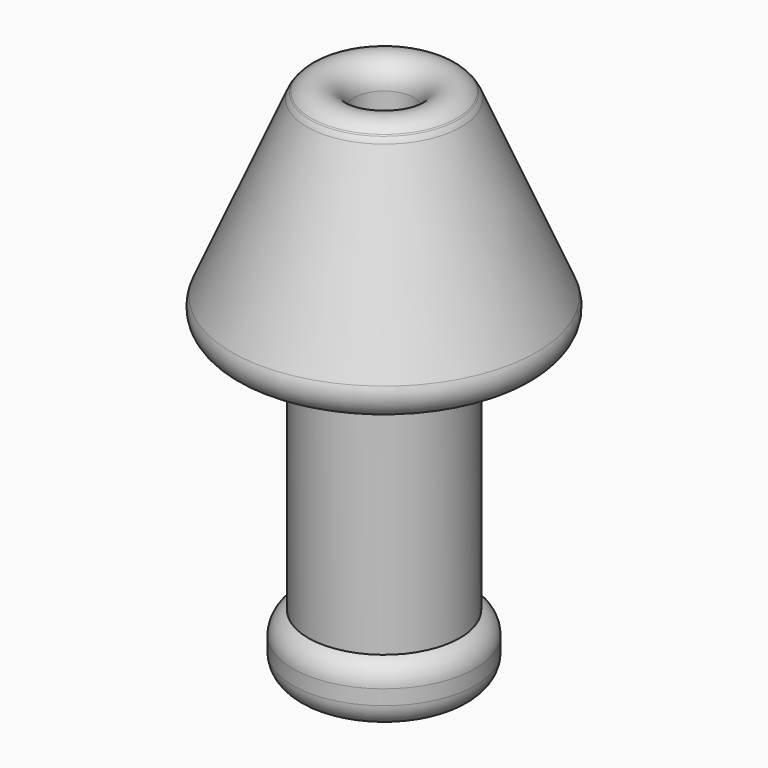
from build123d import *

# Parameters (mm, degrees)
F0_W = 0.5
F0_H = 2


# Not quite as in the source:
# - a fillet or chamfer that OpenCascade refuses, or shapes differently, is made with other operations: its cross-section is extruded or revolved along the edge and cut away or added


with BuildPart() as f1:
    # F0 (on Front) → F1 (revolve)
    with BuildSketch(Plane.XZ):
        Polygon((-2.5, 0), (-1, 0), (-1, 18.7049116939), (-2.5, 16.9229302555), (-5.5, 10), (-2.5, 10), (-2.5, 2), align=None)
        with Locations((-2.75, 1)):
            Rectangle(F0_W, F0_H)
    revolve(axis=Axis((0, 0, 13.3904740214), (0, 0, 1)))

    # F2: fillet of radius 0.8 on 5 edges, made by hand

    # F2_s1 → F2_t2 (revolve, cut)
    with BuildSketch(Plane.XZ):
        with BuildLine():
            ThreePointArc((-2.424695214, 17.0126243355), (-2.4928760132, 16.918520212), (-2.546704077, 16.8155311495))
            Line((-2.546704077, 16.8155311495), (-2.5613849178, 16.821892982))
            ThreePointArc((-2.5613849178, 16.821892982), (-2.5379640629, 16.8755627139), (-2.5146808408, 16.929292088))
            Line((-2.5146808408, 16.929292088), (-2.5122406636, 16.9332339517))
            ThreePointArc((-2.5122406636, 16.9332339517), (-2.4745308925, 16.9780326932), (-2.4369358776, 17.0229280317))
            Line((-2.4369358776, 17.0229280317), (-2.424695214, 17.0126243355))
        make_face()
    revolve(axis=Axis((0, 0, 16.9229302555), (0, 0, 1)), mode=Mode.SUBTRACT)

    # F2_s3 → F2_t4 (revolve, cut)
    with BuildSketch(Plane.XZ):
        with BuildLine():
            ThreePointArc((-5.0157118449, 11.1179416236), (-4.9504273448, 10.3608017674), (-4.2816698032, 9.99985))
            Line((-4.2816698032, 9.99985), (-4.2816698032, 9.98385))
            ThreePointArc((-4.2816698032, 9.98385), (-4.8908349016, 9.984), (-5.5, 9.984))
            Line((-5.5, 9.984), (-5.5146808408, 10.0063618325))
            ThreePointArc((-5.5146808408, 10.0063618325), (-5.2724679468, 10.5653028232), (-5.0303926857, 11.1243034561))
            Line((-5.0303926857, 11.1243034561), (-5.0157118449, 11.1179416236))
        make_face()
    revolve(axis=Axis((0, 0, 10), (0, 0, 1)), mode=Mode.SUBTRACT)

    # F2_s5 → F2_t6 (revolve, cut)
    with BuildSketch(Plane.XZ):
        with BuildLine():
            ThreePointArc((-0.99985, 16.5126600652), (-1.5256480152, 17.2642006639), (-2.4118831788, 17.0278448749))
            Line((-2.4118831788, 17.0278448749), (-2.4241238423, 17.0381485711))
            ThreePointArc((-2.4241238423, 17.0381485711), (-1.7181248748, 17.876633682), (-1.0122406636, 18.7152153901))
            Line((-1.0122406636, 18.7152153901), (-0.984, 18.7049116939))
            ThreePointArc((-0.984, 18.7049116939), (-0.984, 17.6087858796), (-0.98385, 16.5126600652))
            Line((-0.98385, 16.5126600652), (-0.99985, 16.5126600652))
        make_face()
    revolve(axis=Axis((0, 0, 18.7049116939), (0, 0, 1)), mode=Mode.SUBTRACT)

    # F2_s7 → F2_t8 (revolve, cut)
    with BuildSketch(Plane.XZ):
        with BuildLine():
            ThreePointArc((-2.5000562324, 2.0001390608), (-2.8634466855, 1.7057368158), (-3.00015, 1.2584812882))
            Line((-3.00015, 1.2584812882), (-3.01615, 1.2584812882))
            ThreePointArc((-3.01615, 1.2584812882), (-3.016, 1.6292406441), (-3.016, 2))
            Line((-3.016, 2), (-3, 2.016))
            ThreePointArc((-3, 2.016), (-2.7500281162, 2.016), (-2.5060543571, 2.0149722163))
            Line((-2.5060543571, 2.0149722163), (-2.5000562324, 2.0001390608))
        make_face()
    revolve(axis=Axis((0, 0, 2), (0, 0, 1)), mode=Mode.SUBTRACT)

    # F2_s9 → F2_t10 (revolve, cut)
    with BuildSketch(Plane.XZ):
        with BuildLine():
            ThreePointArc((-3.00015, 0.79985), (-2.7658354249, 0.2341645751), (-2.20015, -0.00015))
            Line((-2.20015, -0.00015), (-2.20015, -0.01615))
            ThreePointArc((-2.20015, -0.01615), (-2.600075, -0.016), (-3, -0.016))
            Line((-3, -0.016), (-3.016, 0))
            ThreePointArc((-3.016, 0), (-3.016, 0.399925), (-3.01615, 0.79985))
            Line((-3.01615, 0.79985), (-3.00015, 0.79985))
        make_face()
    revolve(axis=Axis((0, 0, 0), (0, 0, 1)), mode=Mode.SUBTRACT)


solid = f1.part
